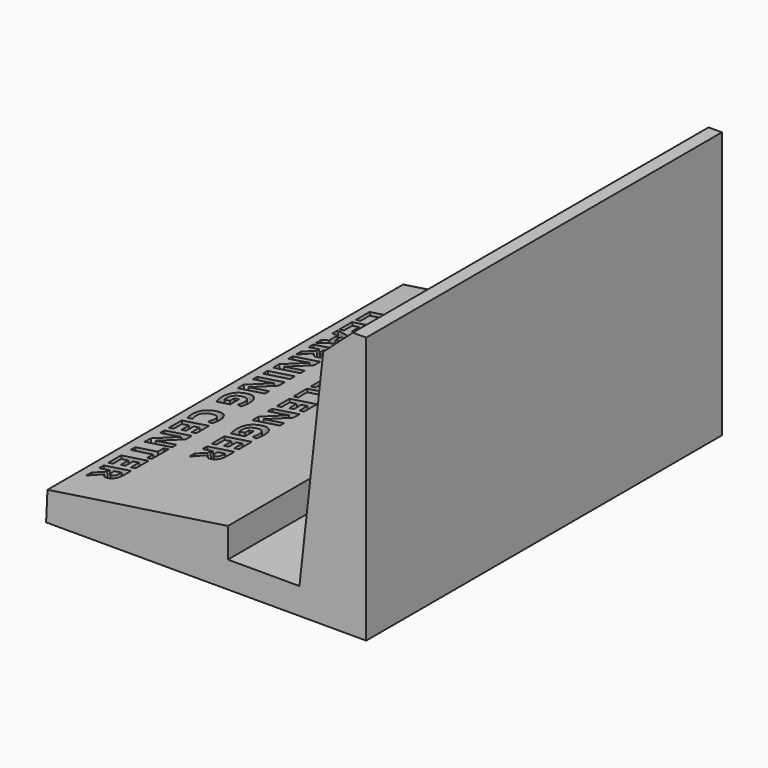
from build123d import *

# Parameters (mm, degrees)
F1_DEPTH     = 63.5
F2_TEXT_SIZE = 5.53941451
F3_DEPTH     = 1.778
F4_W         = 3.175
F4_H         = 5.334
F5_DEPTH     = 38.101
F6_SIZE      = 3.81


# Not quite as in the source:
# - Text() gives the source's letters only with a copy of the font that has no kerning and outlines rounded to 1/6400 em; it was checked with that copy


with BuildPart() as f1:
    # F0 (on Front) → F1 (new body)
    with BuildSketch(Plane.XZ):
        Polygon((6.8806437775, -13.3767249063), (-18.8883699325, -17.2129982766), (-19.0880340623, -21.3787152052), (26.6319659377, -21.3787152052), (26.6319659377, 16.7212847948), (20.9128540009, 16.7212847948), (17.0937336778, -17.6146730453), (6.8806437775, -17.6146730453), align=None)
    extrude(amount=F1_DEPTH)

    # F2 (on face) → F3 (cut)
    with BuildSketch(Plane(origin=(2.0974232414, 0, -14.0888104278), x_dir=(0.9890994867, 0, 0.1472487874), z_dir=(-0.1472487874, 0, 0.9890994867))):
        with Locations(Location((-12.1789461583, -13.1238807396), (0, 0, -90))):
            Text('CHALLENGER', F2_TEXT_SIZE, font='Open Sans', font_style=FontStyle.BOLD, text_align=(TextAlign.LEFT, TextAlign.BOTTOM))
        with Locations(Location((-19.7125498918, -7.3663517833), (0, 0, -90))):
            Text('LEARNING CENTER', F2_TEXT_SIZE, font='Open Sans', font_style=FontStyle.BOLD, text_align=(TextAlign.LEFT, TextAlign.BOTTOM))
    extrude(amount=-F3_DEPTH, mode=Mode.SUBTRACT)

    # F4 (on face) → F5 (cut, through all)
    with BuildSketch(Plane(origin=(0, 0, -21.3787152052), x_dir=(1, 0, 0), z_dir=(0, 0, -1))):
        with Locations((3.8326437775, 31.75)):
            Rectangle(F4_W, F4_H)
    extrude(amount=-F5_DEPTH, mode=Mode.SUBTRACT)

    # F6
    f6_edges = [f1.edges().sort_by_distance(p)[0] for p in [
        (20.912854, -31.75, 16.721285),
    ]]
    chamfer(f6_edges, length=F6_SIZE)


solid = f1.part
